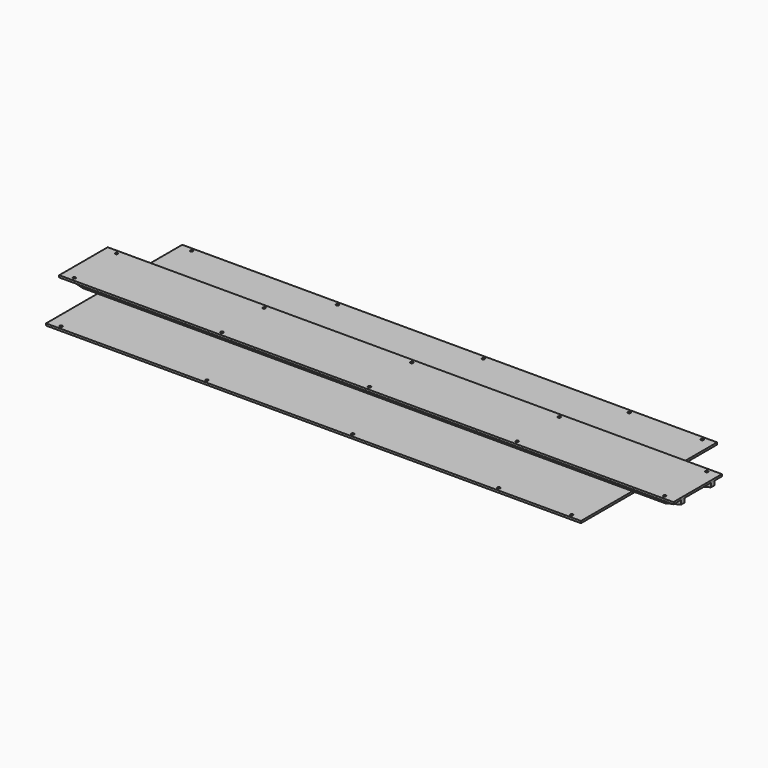
from build123d import *

# Parameters (mm, degrees)
F0_W      = 3352.8
F0_H      = 1066.8
F1_DEPTH  = 12.7
F2_D      = 17.4625
F2_DEPTH  = 50.8
F2_TIP    = 5.2462642799
F4_W      = 3850
F4_H      = 380
F5_DEPTH  = 12.7
F7_D      = 17.4625
F8_W      = 25.4
F8_H      = 50.8
F9_DEPTH  = 3850
F10_SIZE2 = 100
F10_SIZE  = 25
F11_SIZE2 = 100
F11_SIZE  = 25
F12_SIZE2 = 100
F12_SIZE  = 25
F13_SIZE2 = 100
F13_SIZE  = 25


# Not quite as in the source:
# - a length typed as a fraction of an inch, garbled in the dataset ("3 / 203.2 mm" for 3/8 in), is restored


with BuildPart() as f1:
    # F0 (on Top) → F1 (new body)
    with BuildSketch(Plane.XY):
        Rectangle(F0_W, F0_H)
    extrude(amount=F1_DEPTH)

    # F2
    with Locations(Plane(origin=(0, 0, 0), x_dir=(1, 0, 0), z_dir=(0, 0, -1))):
        with Locations((-1600.2, -511.302), (-685.8, -511.302), (228.6, -511.302), (1143, -511.302), (1600.2, -511.302), (1600.2, 511.302), (1143, 511.302), (228.6, 511.302), (-685.8, 511.302), (-1600.2, 511.302)):
            Hole(F2_D / 2, depth=F2_DEPTH)
            with Locations((0, 0, -(F2_DEPTH + F2_TIP / 2))):  # 118° drill point
                Cone(0, F2_D / 2, F2_TIP, mode=Mode.SUBTRACT)


with BuildPart() as f5:
    # F4 (on offset) → F5 (new body)
    with BuildSketch(Plane.XY.offset(76.2)):
        with Locations((56.2, 0)):
            Rectangle(F4_W, F4_H)
    extrude(amount=-F5_DEPTH)

    # F7 (through all)
    with Locations(Plane.XY.offset(76.2)):
        with Locations((-1793.8, 165), (-1793.8, -165), (-868.8, 165), (-868.8, -165), (56.2, 165), (981.2, 165), (56.2, -165), (981.2, -165), (1906.2, 165), (1906.2, -165)):
            Hole(F7_D / 2)


with BuildPart() as f9:
    # F8 (on face) → F9 (new body)
    with BuildSketch(Plane.YZ.offset(1981.2)):
        with Locations((-117.3, 38.1)):
            Rectangle(F8_W, F8_H)
    extrude(amount=-F9_DEPTH)

    # F11
    f11_edges = [f9.edges().sort_by_distance(p)[0] for p in [
        (-1868.8, -117.3, 12.7),
    ]]
    f11_side = f9.faces().sort_by_distance((-1868.8, -117.3, 38.1))[0]
    chamfer(f11_edges, length=F11_SIZE, length2=F11_SIZE2, reference=f11_side)

    # F13
    f13_edges = [f9.edges().sort_by_distance(p)[0] for p in [
        (1981.2, -117.3, 12.7),
    ]]
    f13_side = f9.faces().sort_by_distance((1981.2, -117.3, 38.1))[0]
    chamfer(f13_edges, length=F13_SIZE, length2=F13_SIZE2, reference=f13_side)


with BuildPart() as f9b:
    # F8 (on face) → F9, piece 2 (new body)
    with BuildSketch(Plane.YZ.offset(1981.2)):
        with Locations((117.3, 38.1)):
            Rectangle(F8_W, F8_H)
    extrude(amount=-F9_DEPTH)

    # F10
    f10_edges = [f9b.edges().sort_by_distance(p)[0] for p in [
        (-1868.8, 117.3, 12.7),
    ]]
    f10_side = f9b.faces().sort_by_distance((-1868.8, 117.3, 38.1))[0]
    chamfer(f10_edges, length=F10_SIZE, length2=F10_SIZE2, reference=f10_side)

    # F12
    f12_edges = [f9b.edges().sort_by_distance(p)[0] for p in [
        (1981.2, 117.3, 12.7),
    ]]
    f12_side = f9b.faces().sort_by_distance((1981.2, 117.3, 38.1))[0]
    chamfer(f12_edges, length=F12_SIZE, length2=F12_SIZE2, reference=f12_side)


solid = Compound([f1.part, f5.part, f9.part, f9b.part])
